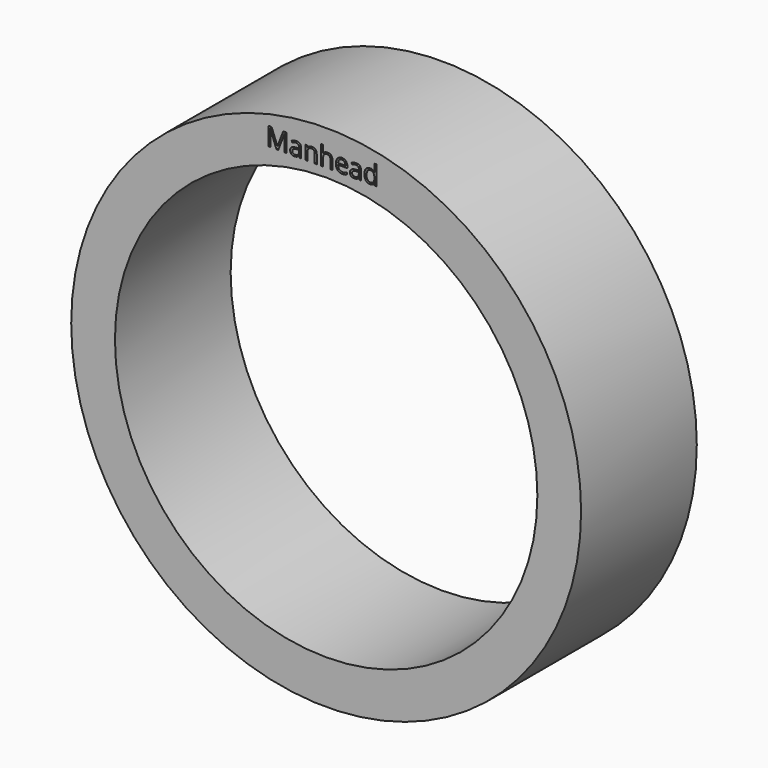
from build123d import *

# Parameters (mm, degrees)
F0_R         = 35.2547350521
F1_DEPTH     = 20
F2_R         = 29.2061643966
F3_DEPTH     = 20.001
F4_TEXT_SIZE = 3.5293814209
F5_DEPTH     = 20.001


# Not quite as in the source:
# - Text() gives the source's letters only with a copy of the font that has no kerning and outlines rounded to 1/6400 em; it was checked with that copy


with BuildPart() as f1:
    # F0 (on Front) → F1 (new body)
    with BuildSketch(Plane.XZ):
        Circle(F0_R)
    extrude(amount=-F1_DEPTH)

    # F2 (on face) → F3 (cut, through all)
    with BuildSketch(Plane.XZ):
        Circle(F2_R)
    extrude(amount=-F3_DEPTH, mode=Mode.SUBTRACT)

    # F4 (on Front) → F5 (cut, through all)
    with BuildSketch(Plane.XZ):
        with Locations((-8.3305025473, 30.3895883262)):
            Text('Manhead', F4_TEXT_SIZE, font='Open Sans', text_align=(TextAlign.LEFT, TextAlign.BOTTOM))
    extrude(amount=-F5_DEPTH, mode=Mode.SUBTRACT)


solid = f1.part
